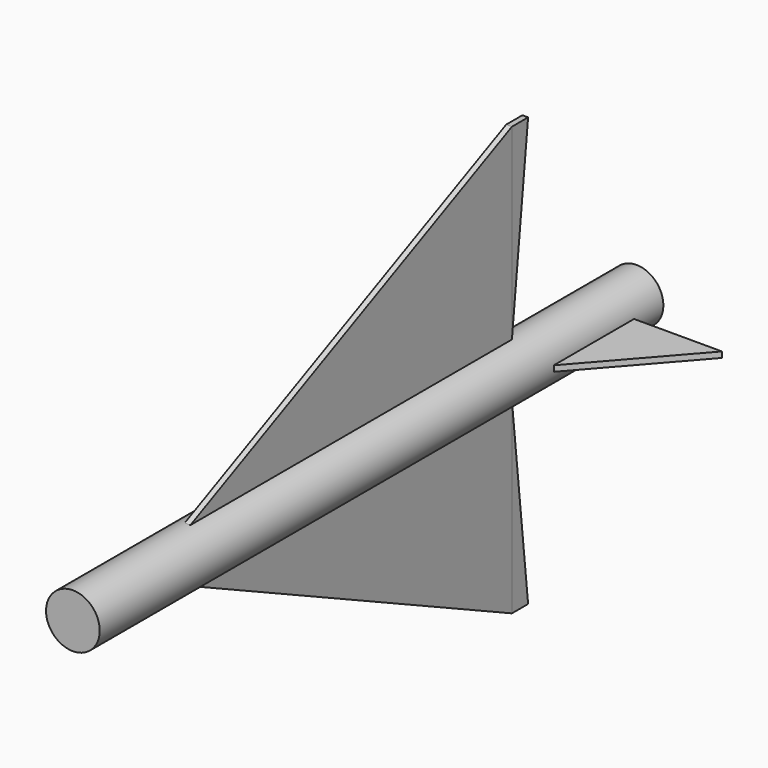
from build123d import *

# Parameters (mm, degrees)
F0_R      = 936
F3_DEPTH  = 14012
F4_DEPTH  = 100
F5_DEPTH  = 100
F6_DEPTH  = 5000
F7_DEPTH  = 5557
F11_DEPTH = 100


# Not quite as in the source:
# - the program builds the solid bodies; features that only make, move or delete a surface that nothing else refers to are left out


with BuildPart() as f3:
    # F0 (on Front) → F3 (new body)
    with BuildSketch(Plane.XZ):
        Circle(F0_R)
    extrude(amount=-F3_DEPTH)

    # F6 (add): a face of the model
    f6_faces = [f3.faces().sort_by_distance(p)[0] for p in [
        (0, 0, 0),
    ]]
    extrude(f6_faces, amount=F6_DEPTH)

    # F7 (add): a face of the model
    f7_faces = [f3.faces().sort_by_distance(p)[0] for p in [
        (0, 14012, 0),
    ]]
    extrude(f7_faces, amount=F7_DEPTH)


with BuildPart() as f4:
    # F1 (on Right) → F4 (new body, symmetric)
    with BuildSketch(Plane.YZ):
        Polygon((14012, 7470), (0, 936), (14012, 936), align=None)
    extrude(amount=F4_DEPTH, both=True)


with BuildPart() as f4b:
    # F1 (on Right) → F4, piece 2 (new body, symmetric)
    with BuildSketch(Plane.YZ):
        Polygon((14012, -7470), (14012, -936), (0, -936), align=None)
    extrude(amount=F4_DEPTH, both=True)


with BuildPart() as f5:
    # F2 (on Right) → F5 (new body, symmetric)
    with BuildSketch(Plane.YZ):
        Polygon((14718, 7470), (14012, 7470), (14012, 936), align=None)
    extrude(amount=F5_DEPTH, both=True)


with BuildPart() as f5b:
    # F2 (on Right) → F5, piece 2 (new body, symmetric)
    with BuildSketch(Plane.YZ):
        Polygon((14718, -7470), (14012, -936), (14012, -7470), align=None)
    extrude(amount=F5_DEPTH, both=True)


with BuildPart() as f11:
    # F10 (on Top) → F11 (new body, symmetric)
    with BuildSketch(Plane.XY):
        Polygon((936, 14791.109085083), (4000, 18291.109085083), (936, 18291.109085083), align=None)
    extrude(amount=F11_DEPTH, both=True)


solid = Compound([f3.part, f4.part, f4b.part, f5.part, f5b.part, f11.part])
